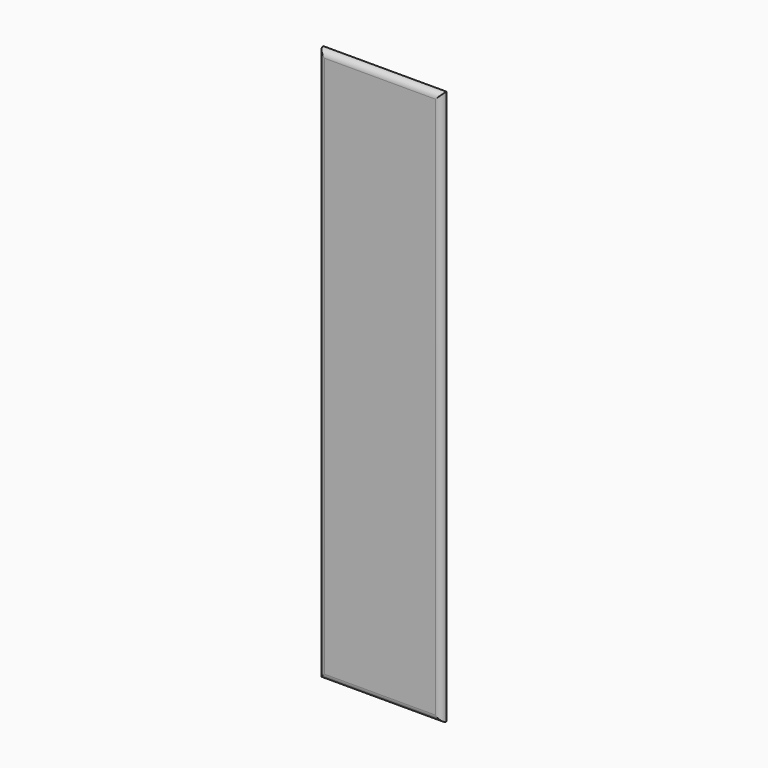
from build123d import *

# Parameters (mm, degrees)
F0_W     = 400
F0_H     = 1800
F1_DEPTH = 20
F2_R     = 19.99999


# Not quite as in the source:
# - a fillet or chamfer is up to 0.001 mm smaller than in the source, because OpenCascade refuses the exact size


with BuildPart() as f1:
    # F0 (on Front) → F1 (new body)
    with BuildSketch(Plane.XZ):
        with Locations((-251.3578593976, -15.0474123657)):
            Rectangle(F0_W, F0_H)
    extrude(amount=F1_DEPTH)

    # F2 (radius 20 in the source; OpenCascade refuses exactly that, so slightly less here)
    f2_edges = [f1.edges().sort_by_distance(p)[0] for p in [
        (-251.357859, -20, -915.047412),
        (-451.357859, -20, -15.047412),
        (-251.357859, -20, 884.952588),
        (-51.357859, -20, -15.047412),
    ]]
    fillet(f2_edges, radius=F2_R)


solid = f1.part
